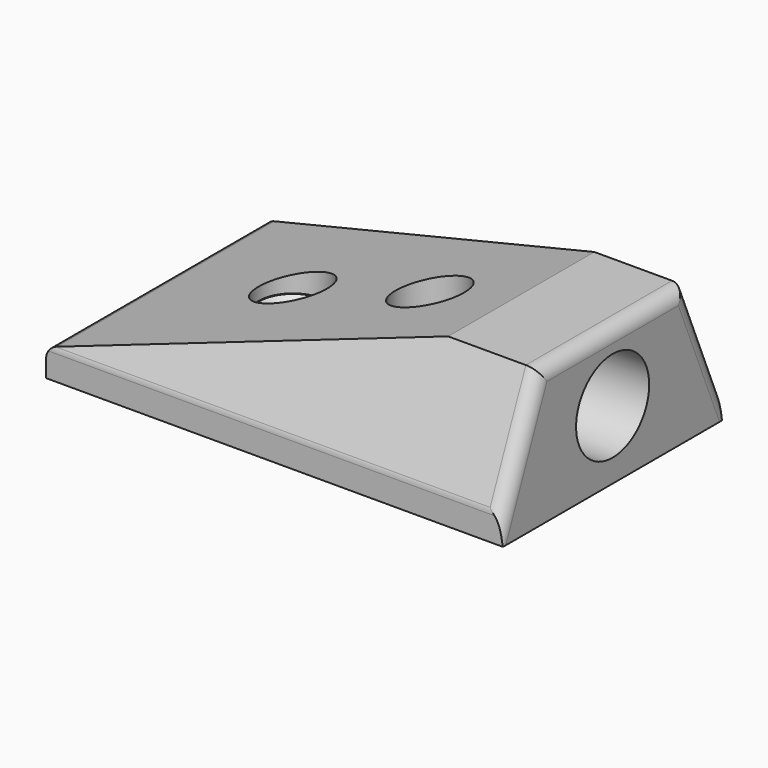
from build123d import *

# Parameters (mm, degrees)
F0_W        = 50
F0_H        = 30
F1_DEPTH    = 15
F2_SIZE2    = 12
F2_SIZE     = 40
F3_C1_SIZE2 = 5
F3_C1_SIZE  = 12
F3_C2_SIZE2 = 12
F3_C2_SIZE  = 5
F5_T1_DEPTH = 35.5802298817
F5_T3_DEPTH = 52.025
F5_T5_DEPTH = 27.5
F5_T7_DEPTH = 20.5
F5_T9_DEPTH = 20.5
F6_R        = 5
F7_DEPTH    = 10
F8_R        = 2.5
F8_R_2      = 2.6409986757
F9_DEPTH    = 40
F10_R       = 3.75
F11_DEPTH   = 10
F12_SIZE    = 1


# Not quite as in the source:
# - a fillet or chamfer that OpenCascade refuses, or shapes differently, is made with other operations: its cross-section is extruded or revolved along the edge and cut away or added
# - two fillets or chamfers of one size are made in one step


with BuildPart() as f1:
    # F0 (on Top) → F1 (new body)
    with BuildSketch(Plane.XY):
        with Locations((-15, 0)):
            Rectangle(F0_W, F0_H)
    extrude(amount=F1_DEPTH)

    # F2
    f2_edges = [f1.edges().sort_by_distance(p)[0] for p in [
        (-40, 0, 15),
    ]]
    f2_side = f1.faces().sort_by_distance((-15, 0, 15))[0]
    chamfer(f2_edges, length=F2_SIZE, length2=F2_SIZE2, reference=f2_side)

    # F3: chamfer of 12 x 5 on 2 edges, made by hand

    # F3_c1
    f3_c1_edges = [f1.edges().sort_by_distance(p)[0] for p in [
        (5, 15, 15),
    ]]
    f3_c1_side = f1.faces().sort_by_distance((5, 15, 14.9))[0]
    chamfer(f3_c1_edges, length=F3_C1_SIZE, length2=F3_C1_SIZE2, reference=f3_c1_side)

    # F3_c2
    f3_c2_edges = [f1.edges().sort_by_distance(p)[0] for p in [
        (5, -15, 15),
    ]]
    f3_c2_side = f1.faces().sort_by_distance((5, -14.9, 15))[0]
    chamfer(f3_c2_edges, length=F3_C2_SIZE, length2=F3_C2_SIZE2, reference=f3_c2_side)

    # F5: fillet of radius 1.5 on 6 edges, made by hand

    # F5_s2 → F5_t1 (cut)
    with BuildSketch(Plane.XZ.offset(-17.7901149408)):
        with BuildLine():
            ThreePointArc((-38.9310218283, 3.3206934515), (-39.7034393924, 2.7793498181), (-40, 1.8839540237))
            Line((-40, 1.8839540237), (-40, 3))
            Line((-40, 3), (-38.9310218283, 3.3206934515))
        make_face()
    extrude(amount=F5_T1_DEPTH, mode=Mode.SUBTRACT)

    # F5_s4 → F5_t3 (cut)
    with BuildSketch(Plane.YZ.offset(-41.275)):
        with BuildLine():
            ThreePointArc((14.8846153846, 3.2769230769), (14.9708710135, 2.9941742027), (15, 2.7))
            Line((15, 2.7), (15, 3))
            Line((15, 3), (14.8846153846, 3.2769230769))
        make_face()
        with BuildLine():
            ThreePointArc((-14.8846153846, 3.2769230769), (-14.9708710135, 2.9941742027), (-15, 2.7))
            Line((-15, 2.7), (-15, 3))
            Line((-15, 3), (-14.8846153846, 3.2769230769))
        make_face()
    extrude(amount=F5_T3_DEPTH, mode=Mode.SUBTRACT)

    # F5_s6 → F5_t5 (cut)
    with BuildSketch(Plane.XZ.offset(-13.75)):
        with BuildLine():
            ThreePointArc((10, 13.5), (9.5606601718, 14.5606601718), (8.5, 15))
            Line((8.5, 15), (10, 15))
            Line((10, 15), (10, 13.5))
        make_face()
    extrude(amount=F5_T5_DEPTH, mode=Mode.SUBTRACT)

    # F5_s8 → F5_t7 (cut)
    with BuildSketch(Plane(origin=(0, 2.5961538462, -6.2307692308), x_dir=(1, 0, 0), z_dir=(0, -0.3846153846, 0.9230769231))):
        with BuildLine():
            ThreePointArc((10, 13.5), (9.5606601718, 14.5606601718), (8.5, 15))
            Line((8.5, 15), (10, 15))
            Line((10, 15), (10, 13.5))
        make_face()
    extrude(amount=F5_T7_DEPTH, mode=Mode.SUBTRACT)

    # F5_s10 → F5_t9 (cut)
    with BuildSketch(Plane(origin=(0, 5.2884615385, 12.6923076923), x_dir=(1, 0, 0), z_dir=(0, -0.3846153846, -0.9230769231))):
        with BuildLine():
            ThreePointArc((10, 13.5), (9.5606601718, 14.5606601718), (8.5, 15))
            Line((8.5, 15), (10, 15))
            Line((10, 15), (10, 13.5))
        make_face()
    extrude(amount=F5_T9_DEPTH, mode=Mode.SUBTRACT)

    # F6 (on face) → F7 (cut)
    with BuildSketch(Plane.YZ.offset(10)):
        with Locations((0, 7.5)):
            Circle(F6_R)
    extrude(amount=-F7_DEPTH, mode=Mode.SUBTRACT)

    # F8 (on face) → F9 (cut)
    with BuildSketch(Plane(origin=(0, 0, 0), x_dir=(1, 0, 0), z_dir=(0, 0, -1))):
        with Locations((-10, 0)):
            Circle(F8_R)
        with Locations((-25, 0)):
            Circle(F8_R_2)
    extrude(amount=-F9_DEPTH, mode=Mode.SUBTRACT)

    # F10 (on face) → F11 (cut)
    with BuildSketch(Plane.XY.offset(15)):
        with Locations((-10, 0)):
            Circle(F10_R)
        with Locations((-25, 0)):
            Circle(F10_R)
    extrude(amount=-F11_DEPTH, mode=Mode.SUBTRACT)

    # F12
    f12_edges = [f1.edges().sort_by_distance(p)[0] for p in [
        (-27.640999, 0, 5),
        (-12.5, 0, 5),
    ]]
    chamfer(f12_edges, length=F12_SIZE)


solid = f1.part
